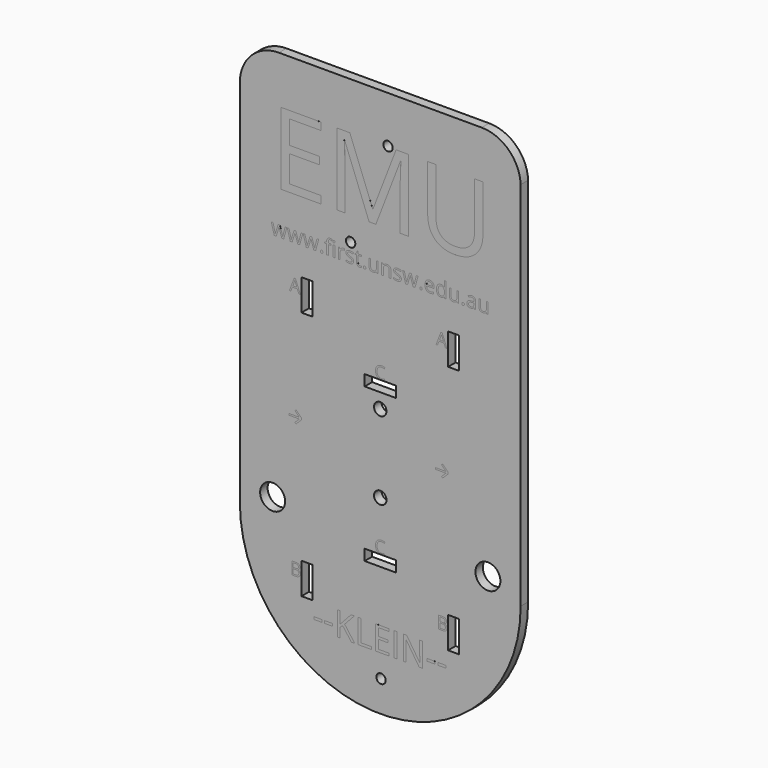
from build123d import *

# Parameters (mm, degrees)
F0_W            = 90
F0_H            = 135
F1_DEPTH        = 3
F2_W            = 10
F2_H            = 3.5
F2_W_2          = 3.5
F2_H_2          = 10
F3_DEPTH        = 25
F4_R            = 4
F5_DEPTH        = 25
F6_R            = 1.5
F7_DEPTH        = 25
F8_R            = 1.5
F8_R_2          = 2
F9_DEPTH        = 25
F10_TEXT_SIZE   = 5.5555555556
F10_TEXT_SIZE_2 = 6.5747956383
F10_TEXT_SIZE_3 = 32.3933477946
F10_TEXT_SIZE_4 = 10.7877707599
F11_DEPTH       = 0.001


# Not quite as in the source:
# - a feature names something its author has since deleted; it is built from what else it names
# - Text() gives the source's letters only with a copy of the font that has no kerning and outlines rounded to 1/6400 em; it was checked with that copy


with BuildPart() as f1:
    # F0 (on Front) → F1 (new body)
    with BuildSketch(Plane.XZ):
        with Locations((-45, 67.5)):
            Rectangle(F0_W, F0_H)
        with BuildLine():
            ThreePointArc((-90, 0), (-45, -45), (0, 0))
            Line((0, 0), (-90, 0))
        make_face()
    extrude(amount=F1_DEPTH)

    # F2 (on face) → F3 (cut)
    with BuildSketch(Plane.XZ.offset(3)):
        with Locations((-45, 47.5)):
            Rectangle(F2_W, F2_H)
        with Locations((-21.5, 65)):
            Rectangle(F2_W_2, F2_H_2)
        with Locations((-68.5, 65)):
            Rectangle(F2_W_2, F2_H_2)
        with Locations((-45, -1.75)):
            Rectangle(F2_W, F2_H)
        with Locations((-68.5, -15)):
            Rectangle(F2_W_2, F2_H_2)
        with Locations((-21.5, -15)):
            Rectangle(F2_W_2, F2_H_2)
    extrude(amount=-F3_DEPTH, mode=Mode.SUBTRACT)

    # F4 (on face) → F5 (cut)
    with BuildSketch(Plane.XZ.offset(3)):
        with Locations((-10.5, 5)):
            Circle(F4_R)
        with Locations((-79.5, 5)):
            Circle(F4_R)
    extrude(amount=-F5_DEPTH, mode=Mode.SUBTRACT)

    # F6 (on face) → F7 (cut)
    with BuildSketch(Plane.XZ.offset(3)):
        with Locations((-44.75, -35)):
            Circle(F6_R)
        with BuildLine():
            ThreePointArc((-12.5, 131), (-3.82947654, 127.5077290138), (0, 118.9807692308))
            Line((0, 118.9807692308), (0, 135))
            Line((0, 135), (-90, 135))
            Line((-90, 135), (-90, 118.9807692308))
            ThreePointArc((-90, 118.9807692308), (-86.17052346, 127.5077290138), (-77.5, 131))
            Line((-77.5, 131), (-12.5, 131))
        make_face()
    extrude(amount=-F7_DEPTH, mode=Mode.SUBTRACT)

    # F8 (on face) → F9 (cut)
    with BuildSketch(Plane.XZ.offset(3)):
        with Locations((-54.5, 85)):
            Circle(F8_R)
        with Locations((-42.5, 116)):
            Circle(F8_R)
        with Locations((-45, 41)):
            Circle(F8_R_2)
        with Locations((-45, 16)):
            Circle(F8_R_2)
    extrude(amount=-F9_DEPTH, mode=Mode.SUBTRACT)

    # F10 (on face) → F11 (join)
    with BuildSketch(Plane.XZ.offset(3)):
        with Locations((-46.8498263889, 0.1)):
            Text('C', F10_TEXT_SIZE, font='Open Sans', text_align=(TextAlign.LEFT, TextAlign.BOTTOM))
        with Locations((-73.9046458333, -15)):
            Text('B', F10_TEXT_SIZE, font='Open Sans', text_align=(TextAlign.LEFT, TextAlign.BOTTOM))
        with Locations((-26.9046458333, -15)):
            Text('B', F10_TEXT_SIZE, font='Open Sans', text_align=(TextAlign.LEFT, TextAlign.BOTTOM))
        with Locations((-46.8498263889, 49.35)):
            Text('C', F10_TEXT_SIZE, font='Open Sans', text_align=(TextAlign.LEFT, TextAlign.BOTTOM))
        with Locations((-27.1268680556, 65)):
            Text('A', F10_TEXT_SIZE, font='Open Sans', text_align=(TextAlign.LEFT, TextAlign.BOTTOM))
        with Locations((-74.1268680556, 65)):
            Text('A', F10_TEXT_SIZE, font='Open Sans', text_align=(TextAlign.LEFT, TextAlign.BOTTOM))
        with Locations((-80, 78.9429367283)):
            Text('www.first.unsw.edu.au', F10_TEXT_SIZE_2, font='Open Sans', text_align=(TextAlign.LEFT, TextAlign.BOTTOM))
        with Locations((-80, 92.6767895879)):
            Text('EMU', F10_TEXT_SIZE_3, font='Open Sans', text_align=(TextAlign.LEFT, TextAlign.BOTTOM))
        Polygon((-25, 28), (-23.25, 29.75), (-23.25, 30.25), (-25, 32), (-25.3535533906, 31.6464466094), (-23.9571067812, 30.25), (-27.25, 30.25), (-27.25, 29.75), (-23.9571067812, 29.75), (-25.3535533906, 28.3535533906), align=None)
        Polygon((-74.25, 30.25), (-74.25, 29.75), (-70.9571067812, 29.75), (-72.3535533906, 28.3535533906), (-72, 28), (-70.25, 29.75), (-70.25, 30.25), (-72, 32), (-72.3535533906, 31.6464466094), (-70.9571067812, 30.25), align=None)
        with Locations((-66.75, -27.7671949471)):
            Text('--KLEIN--', F10_TEXT_SIZE_4, font='Open Sans', text_align=(TextAlign.LEFT, TextAlign.BOTTOM))
    extrude(amount=F11_DEPTH)


solid = f1.part
